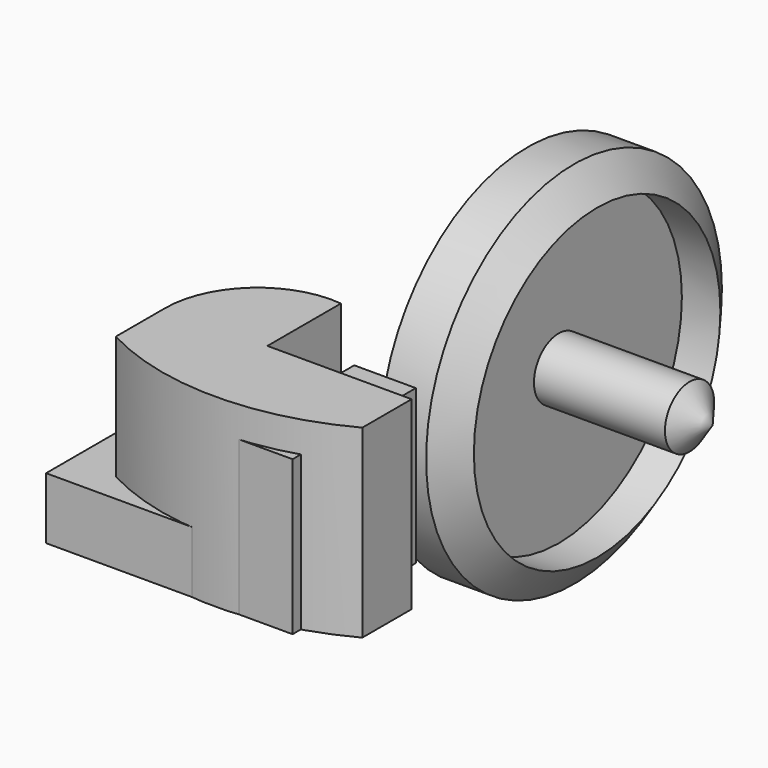
from build123d import *

# Parameters (mm, degrees)
F2_DEPTH = 60
F5_DEPTH = 50
F4_W     = 60
F4_H     = 50
F6_DEPTH = 20


with BuildPart() as f2:
    # F1 (on Top) → F2 (new body)
    with BuildSketch(Plane.XY):
        with BuildLine():
            Line((-31.8526111987, -39.1376554476), (-31.8526111987, -9.3087305754))
            ThreePointArc((-31.8526111987, -9.3087305754), (-55.1020833547, -16.8219917846), (-65.0518675135, -39.1376554476))
            Line((-65.0518675135, -39.1376554476), (-65.0518675135, -59.1376554476))
            ThreePointArc((-65.0518675135, -59.1376554476), (-25.0518675135, -69.1376554476), (14.9481324865, -59.1376554476))
            Line((14.9481324865, -59.1376554476), (14.9481324865, -39.1376554476))
            Line((14.9481324865, -39.1376554476), (-31.8526111987, -39.1376554476))
        make_face()
    extrude(amount=F2_DEPTH)


with BuildPart() as f3:
    # F0 (on Top) → F3 (revolve)
    with BuildSketch(Plane.XY):
        Polygon((-33.5372266173, 147.348228097), (-48.5372266173, 147.348228097), (-48.5372266173, 87.348228097), (11.4627733827, 87.348228097), (3.9627733824, 97.348228097), (-38.5372266173, 97.348228097), (-38.5372266173, 137.348228097), (-26.0372266173, 137.348228097), align=None)
    revolve(axis=Axis((-18.5372266173, 87.348228097, 0), (1, 0, 0)))


with BuildPart() as f5:
    # F4 (on Top) → F5 (new body)
    with BuildSketch(Plane.XY):
        Polygon((-20.023245162, -18.7104548417), (-20.023245162, -68.7104548417), (-0.023245162, -68.7104548417), (-0.023245162, -58.7104548417), (-8.023245162, -58.7104548417), (-8.023245162, -28.7104548417), (-0.023245162, -28.7104548417), (-0.023245162, -18.7104548417), align=None)
    extrude(amount=F5_DEPTH)

    # F4 (on Top) → F6 (join)
    with BuildSketch(Plane.XY):
        with Locations((-50.023245162, -43.7104548417)):
            Rectangle(F4_W, F4_H)
    extrude(amount=F6_DEPTH)


solid = Compound([f2.part, f3.part, f5.part])
